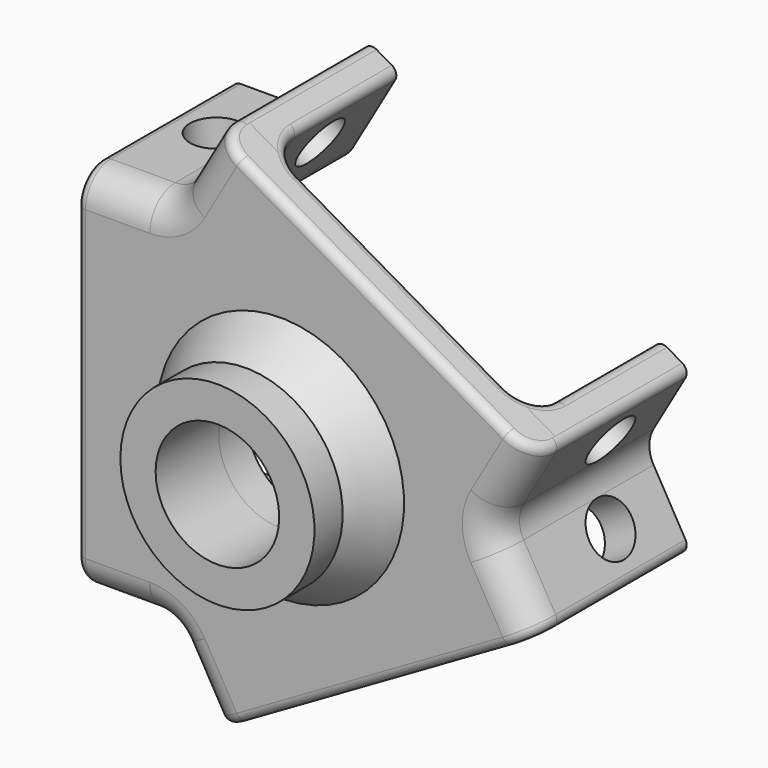
from build123d import *

# Parameters (mm, degrees)
F1_DEPTH      = 10
F6_DEPTH      = 45
F4_W          = 10
F4_H          = 10
F8_R          = 7.5
F11_DEPTH     = 150
F10_R         = 7.5
F12_DEPTH     = 120
F9_R          = 7.5
F13_DEPTH     = 120
F14_R         = 9
F15_T1_DEPTH  = 87
F15_T3_DEPTH  = 67
F15_T5_DEPTH  = 42.25
F15_T7_DEPTH  = 52.25
F15_T9_DEPTH  = 67
F15_T11_DEPTH = 87
F15_T13_DEPTH = 87
F15_T15_DEPTH = 67
F15_T18_ANGLE = 90
F15_T20_ANGLE = 90
F15_T22_ANGLE = 90
F15_T24_ANGLE = 90
F15_T26_ANGLE = 90
F15_T28_ANGLE = 90
F15_T30_ANGLE = 90
F15_T32_ANGLE = 90
F15_T34_ANGLE = 90
F15_T36_ANGLE = 90
F15_T38_ANGLE = 90
F15_T40_ANGLE = 90
F16_DEPTH     = 25


# Not quite as in the source:
# - a fillet or chamfer that OpenCascade refuses, or shapes differently, is made with other operations: its cross-section is extruded or revolved along the edge and cut away or added


with BuildPart() as f1:
    # F0 (on Front) → F1 (new body)
    with BuildSketch(Plane.XZ):
        Polygon((-59.0086988402, 78.9222342521), (-84.9086988402, 78.9222342521), (-84.9086988402, -26.0777657479), (-59.0086988402, -26.0777657479), (-46.1141988402, -48.4116948861), (44.8184685572, 4.0883051139), (31.9239685572, 26.4222342521), (44.8184685572, 48.7561633903), (-46.1141988402, 101.2561633903), align=None)
    extrude(amount=-F1_DEPTH)

    # F5 (on face) → F6 (join)
    with BuildSketch(Plane(origin=(0, 10, 0), x_dir=(-1, 0, 0), z_dir=(0, 1, 0))):
        Polygon((37.4539448024, -43.4116948861), (46.1141988402, -48.4116948861), (59.0086988402, -26.0777657479), (84.9086988402, -26.0777657479), (84.9086988402, -16.0777657479), (53.2351961483, -16.0777657479), align=None)
        Polygon((-44.8184685572, 4.0883051139), (-36.1582145193, -0.9116948861), (-20.3769631734, 26.4222342521), (-36.1582145193, 53.7561633903), (-44.8184685572, 48.7561633903), (-31.9239685572, 26.4222342521), align=None)
        Polygon((53.2351961483, 68.9222342521), (84.9086988402, 68.9222342521), (84.9086988402, 78.9222342521), (59.0086988402, 78.9222342521), (46.1141988402, 101.2561633903), (37.4539448024, 96.2561633903), align=None)
    extrude(amount=F6_DEPTH)

    # F4 (on line) → F7 (revolve)
    with BuildSketch(Plane(origin=(-9.1182087742, 0, -5.2644002903), x_dir=(0, -1, 0), z_dir=(-0.8660254038, 0, -0.5))):
        with Locations((17.361, 13.5863541796)):
            Rectangle(F4_W, F4_H)
        Polygon((12.361, 8.5863541796), (12.361, 18.5863541796), (0, 18.5863541796), (0, 1.0863541796), align=None)
    revolve(axis=Axis((-27.161385864, -39.4499748945, 25.9872991592), (0, -1, 0)))

    # F8 (on face) → F11 (cut)
    with BuildSketch(Plane(origin=(-78.430854023, 0, 45.282074683), x_dir=(0, -1, 0), z_dir=(-0.8660254038, 0, 0.5))):
        with Locations((-35, 51.6333103656)):
            Circle(F8_R)
    extrude(amount=-F11_DEPTH, mode=Mode.SUBTRACT)

    # F10 (on face) → F12 (cut)
    with BuildSketch(Plane(origin=(-55.548527936, 0, -32.0709575569), x_dir=(0, -1, 0), z_dir=(-0.8660254038, 0, -0.5))):
        with Locations((-35, -5.8686581915)):
            Circle(F10_R)
    extrude(amount=-F12_DEPTH, mode=Mode.SUBTRACT)

    # F9 (on face) → F13 (cut)
    with BuildSketch(Plane.XY.offset(78.9222342521)):
        with Locations((-71.9086988402, 33.2328826189)):
            Circle(F9_R)
    extrude(amount=-F13_DEPTH, mode=Mode.SUBTRACT)

    # F14
    f14_edges = [f1.edges().sort_by_distance(p)[0] for p in [
        (-71.958699, 0, -26.077766),
        (-52.561449, 0, -37.24473),
        (-59.008699, 27.5, -26.077766),
        (-52.561449, 0, 90.089199),
        (-71.958699, 0, 78.922234),
        (-59.008699, 27.5, 78.922234),
        (38.371219, 0, 15.25527),
        (38.371219, 0, 37.589199),
        (31.923969, 27.5, 26.422234),
        (-45.34457, 10, 82.589199),
        (-69.071947, 10, 68.922234),
        (-53.235196, 32.5, 68.922234),
        (-45.34457, 10, -29.74473),
        (-69.071947, 10, -16.077766),
        (-53.235196, 32.5, -16.077766),
        (20.376963, 32.5, 26.422234),
        (28.267589, 10, 12.75527),
        (28.267589, 10, 40.089199),
    ]]
    fillet(f14_edges, radius=F14_R)

    # F15: fillet of radius 2.5 on 30 edges, made by hand

    # F15_s2 → F15_t1 (cut)
    with BuildSketch(Plane.XY.offset(-17.0777657479)):
        with BuildLine():
            ThreePointArc((-84.9086988402, 2.5), (-84.1764657932, 0.732233047), (-82.4086988402, 0))
            Line((-82.4086988402, 0), (-84.9086988402, 0))
            Line((-84.9086988402, 0), (-84.9086988402, 2.5))
        make_face()
    extrude(amount=F15_T1_DEPTH, mode=Mode.SUBTRACT)

    # F15_s4 → F15_t3 (cut)
    with BuildSketch(Plane.XY.offset(-7.0777657479)):
        with BuildLine():
            ThreePointArc((-84.9086988402, 7.5), (-84.1764657932, 9.267766953), (-82.4086988402, 10))
            Line((-82.4086988402, 10), (-84.9086988402, 10))
            Line((-84.9086988402, 10), (-84.9086988402, 7.5))
        make_face()
    extrude(amount=F15_T3_DEPTH, mode=Mode.SUBTRACT)

    # F15_s6 → F15_t5 (cut)
    with BuildSketch(Plane.XZ.offset(-61.25)):
        with BuildLine():
            ThreePointArc((-84.9086988402, 71.4222342521), (-84.1764657932, 69.6544672991), (-82.4086988402, 68.9222342521))
            Line((-82.4086988402, 68.9222342521), (-84.9086988402, 68.9222342521))
            Line((-84.9086988402, 68.9222342521), (-84.9086988402, 71.4222342521))
        make_face()
        with BuildLine():
            ThreePointArc((-84.9086988402, -18.5777657479), (-84.1764657932, -16.8099987949), (-82.4086988402, -16.0777657479))
            Line((-82.4086988402, -16.0777657479), (-84.9086988402, -16.0777657479))
            Line((-84.9086988402, -16.0777657479), (-84.9086988402, -18.5777657479))
        make_face()
        with BuildLine():
            ThreePointArc((-38.7039448024, 94.0910998808), (-38.4541937461, 95.9881474936), (-39.6190083118, 97.5061633903))
            Line((-39.6190083118, 97.5061633903), (-37.4539448024, 96.2561633903))
            Line((-37.4539448024, 96.2561633903), (-38.7039448024, 94.0910998808))
        make_face()
        with BuildLine():
            ThreePointArc((38.3232780288, 52.5061633903), (36.426230416, 52.7559144466), (34.9082145193, 51.5910998808))
            Line((34.9082145193, 51.5910998808), (36.1582145193, 53.7561633903))
            Line((36.1582145193, 53.7561633903), (38.3232780288, 52.5061633903))
        make_face()
        with BuildLine():
            ThreePointArc((38.3232780288, 0.3383051139), (36.426230416, 0.0885540576), (34.9082145193, 1.2533686234))
            Line((34.9082145193, 1.2533686234), (36.1582145193, -0.9116948861))
            Line((36.1582145193, -0.9116948861), (38.3232780288, 0.3383051139))
        make_face()
        with BuildLine():
            ThreePointArc((-39.6190083118, -44.6616948861), (-38.4541937461, -43.1436789894), (-38.7039448024, -41.2466313766))
            Line((-38.7039448024, -41.2466313766), (-37.4539448024, -43.4116948861))
            Line((-37.4539448024, -43.4116948861), (-39.6190083118, -44.6616948861))
        make_face()
    extrude(amount=F15_T5_DEPTH, mode=Mode.SUBTRACT)

    # F15_s8 → F15_t7 (cut)
    with BuildSketch(Plane.XZ.offset(-61.25)):
        with BuildLine():
            ThreePointArc((-43.9491353307, 100.0061633903), (-45.8461829435, 100.2559144466), (-47.3641988402, 99.0910998808))
            Line((-47.3641988402, 99.0910998808), (-46.1141988402, 101.2561633903))
            Line((-46.1141988402, 101.2561633903), (-43.9491353307, 100.0061633903))
        make_face()
        with BuildLine():
            ThreePointArc((42.6534050477, 2.8383051139), (43.8182196134, 4.3563210106), (43.5684685572, 6.2533686234))
            Line((43.5684685572, 6.2533686234), (44.8184685572, 4.0883051139))
            Line((44.8184685572, 4.0883051139), (42.6534050477, 2.8383051139))
        make_face()
        with BuildLine():
            ThreePointArc((-82.4086988402, 78.9222342521), (-84.1764657932, 78.1900012051), (-84.9086988402, 76.4222342521))
            Line((-84.9086988402, 76.4222342521), (-84.9086988402, 78.9222342521))
            Line((-84.9086988402, 78.9222342521), (-82.4086988402, 78.9222342521))
        make_face()
        with BuildLine():
            ThreePointArc((-84.9086988402, -23.5777657479), (-84.1764657932, -25.3455327009), (-82.4086988402, -26.0777657479))
            Line((-82.4086988402, -26.0777657479), (-84.9086988402, -26.0777657479))
            Line((-84.9086988402, -26.0777657479), (-84.9086988402, -23.5777657479))
        make_face()
        with BuildLine():
            ThreePointArc((42.6534050477, 50.0061633903), (43.8182196134, 48.4881474936), (43.5684685572, 46.5910998808))
            Line((43.5684685572, 46.5910998808), (44.8184685572, 48.7561633903))
            Line((44.8184685572, 48.7561633903), (42.6534050477, 50.0061633903))
        make_face()
        with BuildLine():
            ThreePointArc((-43.9491353307, -47.1616948861), (-45.8461829435, -47.4114459424), (-47.3641988402, -46.2466313766))
            Line((-47.3641988402, -46.2466313766), (-46.1141988402, -48.4116948861))
            Line((-46.1141988402, -48.4116948861), (-43.9491353307, -47.1616948861))
        make_face()
    extrude(amount=F15_T7_DEPTH, mode=Mode.SUBTRACT)

    # F15_s10 → F15_t9 (cut)
    with BuildSketch(Plane(origin=(-3.9526692976, 0, 2.282074683), x_dir=(0, 1, 0), z_dir=(-0.8660254038, 0, 0.5))):
        with BuildLine():
            ThreePointArc((7.5, -64.6333103656), (9.267766953, -63.9010773186), (10, -62.1333103656))
            Line((10, -62.1333103656), (10, -64.6333103656))
            Line((10, -64.6333103656), (7.5, -64.6333103656))
        make_face()
    extrude(amount=F15_T9_DEPTH, mode=Mode.SUBTRACT)

    # F15_s12 → F15_t11 (cut)
    with BuildSketch(Plane(origin=(4.7075847403, 0, -2.717925317), x_dir=(0, 1, 0), z_dir=(-0.8660254038, 0, 0.5))):
        with BuildLine():
            ThreePointArc((2.5, -64.6333103656), (0.732233047, -63.9010773186), (0, -62.1333103656))
            Line((0, -62.1333103656), (0, -64.6333103656))
            Line((0, -64.6333103656), (2.5, -64.6333103656))
        make_face()
    extrude(amount=F15_T11_DEPTH, mode=Mode.SUBTRACT)

    # F15_s14 → F15_t13 (cut)
    with BuildSketch(Plane(origin=(-47.7542993019, 0, -27.5709575569), x_dir=(0, 1, 0), z_dir=(0.8660254038, 0, 0.5))):
        with BuildLine():
            ThreePointArc((0, -16.3686581915), (0.732233047, -18.1364251445), (2.5, -18.8686581915))
            Line((2.5, -18.8686581915), (0, -18.8686581915))
            Line((0, -18.8686581915), (0, -16.3686581915))
        make_face()
    extrude(amount=F15_T13_DEPTH, mode=Mode.SUBTRACT)

    # F15_s16 → F15_t15 (cut)
    with BuildSketch(Plane(origin=(-39.0940452641, 0, -22.5709575569), x_dir=(0, 1, 0), z_dir=(0.8660254038, 0, 0.5))):
        with BuildLine():
            ThreePointArc((10, -16.3686581915), (9.267766953, -18.1364251445), (7.5, -18.8686581915))
            Line((7.5, -18.8686581915), (10, -18.8686581915))
            Line((10, -18.8686581915), (10, -16.3686581915))
        make_face()
    extrude(amount=F15_T15_DEPTH, mode=Mode.SUBTRACT)

    # F15_s17 → F15_t18 (revolve, cut)
    with BuildSketch(Plane.XZ.offset(-9)):
        with BuildLine():
            ThreePointArc((-84.9086988402, 76.4222342521), (-84.1764657932, 78.1900012051), (-82.4086988402, 78.9222342521))
            Line((-82.4086988402, 78.9222342521), (-84.9086988402, 78.9222342521))
            Line((-84.9086988402, 78.9222342521), (-84.9086988402, 76.4222342521))
        make_face()
    revolve(axis=Axis((-84.9086988402, 9, 69.9222342521), (1, 0, 0)), revolution_arc=F15_T18_ANGLE, mode=Mode.SUBTRACT)

    # F15_s19 → F15_t20 (revolve, cut)
    with BuildSketch(Plane.XY.offset(-17.0777657479)):
        with BuildLine():
            ThreePointArc((-84.9086988402, 2.5), (-84.1764657932, 0.732233047), (-82.4086988402, 0))
            Line((-82.4086988402, 0), (-84.9086988402, 0))
            Line((-84.9086988402, 0), (-84.9086988402, 2.5))
        make_face()
    revolve(axis=Axis((-84.9086988402, 9, -17.0777657479), (1, 0, 0)), revolution_arc=F15_T20_ANGLE, mode=Mode.SUBTRACT)

    # F15_s21 → F15_t22 (revolve, cut)
    with BuildSketch(Plane.XZ.offset(-19)):
        with BuildLine():
            ThreePointArc((-84.9086988402, 71.4222342521), (-84.1764657932, 69.6544672991), (-82.4086988402, 68.9222342521))
            Line((-82.4086988402, 68.9222342521), (-84.9086988402, 68.9222342521))
            Line((-84.9086988402, 68.9222342521), (-84.9086988402, 71.4222342521))
        make_face()
    revolve(axis=Axis((-84.9086988402, 19, 59.9222342521), (1, 0, 0)), revolution_arc=F15_T22_ANGLE, mode=Mode.SUBTRACT)

    # F15_s23 → F15_t24 (revolve, cut)
    with BuildSketch(Plane.XY.offset(-7.0777657479)):
        with BuildLine():
            ThreePointArc((-84.9086988402, 7.5), (-84.1764657932, 9.267766953), (-82.4086988402, 10))
            Line((-82.4086988402, 10), (-84.9086988402, 10))
            Line((-84.9086988402, 10), (-84.9086988402, 7.5))
        make_face()
    revolve(axis=Axis((-84.9086988402, 19, -7.0777657479), (1, 0, 0)), revolution_arc=F15_T24_ANGLE, mode=Mode.SUBTRACT)

    # F15_s25 → F15_t26 (revolve, cut)
    with BuildSketch(Plane(origin=(4.7075847403, 0, -2.717925317), x_dir=(0, 1, 0), z_dir=(-0.8660254038, 0, 0.5))):
        with BuildLine():
            ThreePointArc((2.5, -64.6333103656), (0.732233047, -63.9010773186), (0, -62.1333103656))
            Line((0, -62.1333103656), (0, -64.6333103656))
            Line((0, -64.6333103656), (2.5, -64.6333103656))
        make_face()
    revolve(axis=Axis((37.0242399231, 9, 53.2561633903), (0.5, 0, 0.8660254038)), revolution_arc=F15_T26_ANGLE, mode=Mode.SUBTRACT)

    # F15_s27 → F15_t28 (revolve, cut)
    with BuildSketch(Plane.XZ.offset(-9)):
        with BuildLine():
            ThreePointArc((-43.9491353307, 100.0061633903), (-45.8461829435, 100.2559144466), (-47.3641988402, 99.0910998808))
            Line((-47.3641988402, 99.0910998808), (-46.1141988402, 101.2561633903))
            Line((-46.1141988402, 101.2561633903), (-43.9491353307, 100.0061633903))
        make_face()
    revolve(axis=Axis((-38.3199702061, 9, 96.7561633903), (0.5, 0, 0.8660254038)), revolution_arc=F15_T28_ANGLE, mode=Mode.SUBTRACT)

    # F15_s29 → F15_t30 (revolve, cut)
    with BuildSketch(Plane(origin=(-3.9526692976, 0, 2.282074683), x_dir=(0, 1, 0), z_dir=(-0.8660254038, 0, 0.5))):
        with BuildLine():
            ThreePointArc((7.5, -64.6333103656), (9.267766953, -63.9010773186), (10, -62.1333103656))
            Line((10, -62.1333103656), (10, -64.6333103656))
            Line((10, -64.6333103656), (7.5, -64.6333103656))
        make_face()
    revolve(axis=Axis((28.3639858853, 19, 58.2561633903), (0.5, 0, 0.8660254038)), revolution_arc=F15_T30_ANGLE, mode=Mode.SUBTRACT)

    # F15_s31 → F15_t32 (revolve, cut)
    with BuildSketch(Plane.XZ.offset(-19)):
        with BuildLine():
            ThreePointArc((-39.6190083118, 97.5061633903), (-38.4541937461, 95.9881474936), (-38.7039448024, 94.0910998808))
            Line((-38.7039448024, 94.0910998808), (-37.4539448024, 96.2561633903))
            Line((-37.4539448024, 96.2561633903), (-39.6190083118, 97.5061633903))
        make_face()
    revolve(axis=Axis((-29.6597161683, 19, 91.7561633903), (0.5, 0, 0.8660254038)), revolution_arc=F15_T32_ANGLE, mode=Mode.SUBTRACT)

    # F15_s33 → F15_t34 (revolve, cut)
    with BuildSketch(Plane(origin=(-47.7542993019, 0, -27.5709575569), x_dir=(0, 1, 0), z_dir=(0.8660254038, 0, 0.5))):
        with BuildLine():
            ThreePointArc((0, -16.3686581915), (0.732233047, -18.1364251445), (2.5, -18.8686581915))
            Line((2.5, -18.8686581915), (0, -18.8686581915))
            Line((0, -18.8686581915), (0, -16.3686581915))
        make_face()
    revolve(axis=Axis((-38.3199702061, 9, -43.9116948861), (0.5, 0, -0.8660254038)), revolution_arc=F15_T34_ANGLE, mode=Mode.SUBTRACT)

    # F15_s35 → F15_t36 (revolve, cut)
    with BuildSketch(Plane(origin=(27.5899108273, 0, 15.9290424431), x_dir=(0, 1, 0), z_dir=(-0.8660254038, 0, -0.5))):
        with BuildLine():
            ThreePointArc((2.5, 18.8686581915), (0.732233047, 18.1364251445), (0, 16.3686581915))
            Line((0, 16.3686581915), (0, 18.8686581915))
            Line((0, 18.8686581915), (2.5, 18.8686581915))
        make_face()
    revolve(axis=Axis((37.0242399231, 9, -0.4116948861), (-0.5, 0, 0.8660254038)), revolution_arc=F15_T36_ANGLE, mode=Mode.SUBTRACT)

    # F15_s37 → F15_t38 (revolve, cut)
    with BuildSketch(Plane(origin=(-39.0940452641, 0, -22.5709575569), x_dir=(0, 1, 0), z_dir=(0.8660254038, 0, 0.5))):
        with BuildLine():
            ThreePointArc((7.5, -18.8686581915), (9.267766953, -18.1364251445), (10, -16.3686581915))
            Line((10, -16.3686581915), (10, -18.8686581915))
            Line((10, -18.8686581915), (7.5, -18.8686581915))
        make_face()
    revolve(axis=Axis((-29.6597161683, 19, -38.9116948861), (0.5, 0, -0.8660254038)), revolution_arc=F15_T38_ANGLE, mode=Mode.SUBTRACT)

    # F15_s39 → F15_t40 (revolve, cut)
    with BuildSketch(Plane(origin=(18.9296567895, 0, 10.9290424431), x_dir=(0, 1, 0), z_dir=(-0.8660254038, 0, -0.5))):
        with BuildLine():
            ThreePointArc((7.5, 18.8686581915), (9.267766953, 18.1364251445), (10, 16.3686581915))
            Line((10, 16.3686581915), (10, 18.8686581915))
            Line((10, 18.8686581915), (7.5, 18.8686581915))
        make_face()
    revolve(axis=Axis((28.3639858853, 19, -5.4116948861), (-0.5, 0, 0.8660254038)), revolution_arc=F15_T40_ANGLE, mode=Mode.SUBTRACT)

    # F16 (cut): a face of the model
    f16_faces = [f1.faces().sort_by_distance(p)[0] for p in [
        (-27.161385864, 0, 25.9872991592),
    ]]
    extrude(f16_faces, amount=-F16_DEPTH, mode=Mode.SUBTRACT)


solid = f1.part
